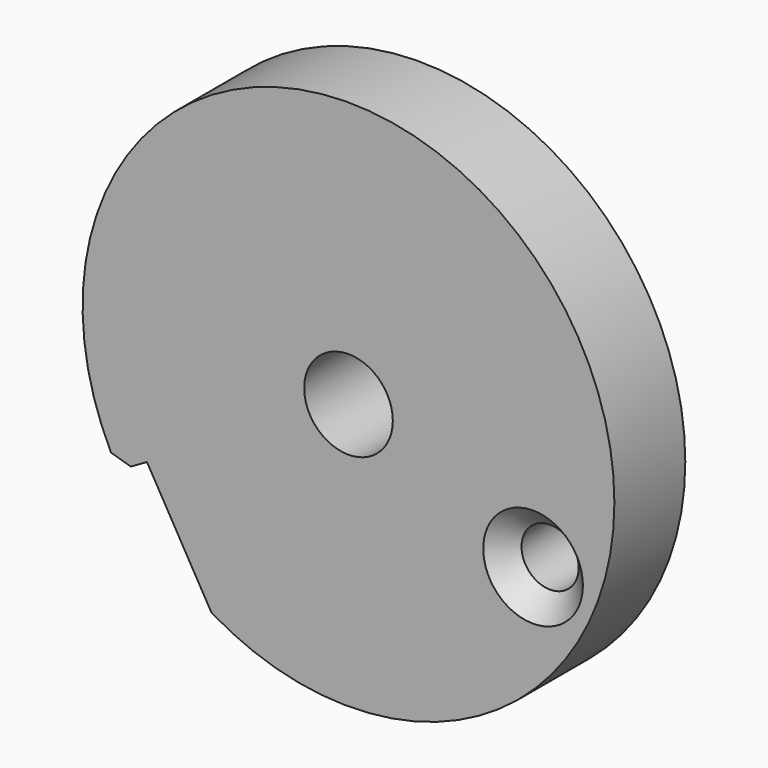
from build123d import *

# Parameters (mm, degrees)
F0_R        = 1.02362
F0_R_2      = 1.5875
F1_DEPTH    = 1.5875
F2_SIZE2    = 0.762
F2_SIZE     = 0.762
F3_T1_DEPTH = 5.9330773534


# Not quite as in the source:
# - a fillet or chamfer that OpenCascade refuses, or shapes differently, is made with other operations: its cross-section is extruded or revolved along the edge and cut away or added


with BuildPart() as f1:
    # F0 (on Front) → F1 (new body, symmetric)
    with BuildSketch(Plane.XZ):
        with BuildLine():
            Line((-6.9308998718, -2.1542398912), (-5.8992384492, -1.5586098912))
            Line((-5.8992384492, -1.5586098912), (-3.5910470257, -5.5565147104))
            ThreePointArc((-3.5910470257, -5.5565147104), (8.1172314393, 9.2773759439), (-6.9308998718, -2.1542398912))
        make_face()
        with Locations((7.9313591488, -0.3737701657)):
            Circle(F0_R, mode=Mode.SUBTRACT)
        with Locations((1.3199729119, 2.6048275917)):
            Circle(F0_R_2, mode=Mode.SUBTRACT)
    extrude(amount=F1_DEPTH, both=True)

    # F2
    f2_edges = [f1.edges().sort_by_distance(p)[0] for p in [
        (6.907739, -1.5875, -0.37377),
    ]]
    chamfer(f2_edges, length=F2_SIZE, length2=F2_SIZE2)

    # F3: chamfer of 0.508 on 1 edges, made by hand

    # F3_s2 → F3_t1 (cut)
    with BuildSketch(Plane.XZ.offset(-2.9665386767)):
        with BuildLine():
            Line((-6.4783627065, -1.892967437), (-7.1860154174, -1.6816380318))
            ThreePointArc((-7.1860154174, -1.6816380318), (-7.0651975677, -1.9134177566), (-6.9308998718, -2.1542398912))
            Line((-6.9308998718, -2.1542398912), (-6.4783627065, -1.892967437))
        make_face()
    extrude(amount=F3_T1_DEPTH, mode=Mode.SUBTRACT)


solid = f1.part
